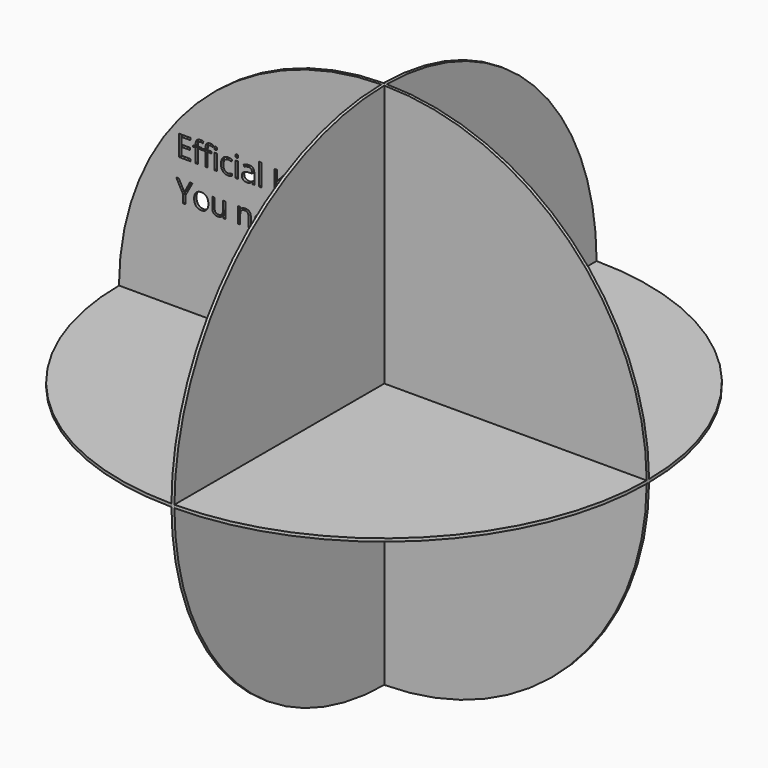
from build123d import *

# Parameters (mm, degrees)
F1_W          = 0.6405815172
F1_H          = 4.2273443089
F1_H_2        = 6.002211788
F2_DEPTH      = 0.4064
F2_DEPTH_BACK = 0.4064
F4_DEPTH      = 0.4064
F4_DEPTH_BACK = 0.4064
F6_DEPTH      = 0.4064
F6_DEPTH_BACK = 0.4064


# Not quite as in the source:
# - a variable given as a bare number and used for a length is read in inches; the dataset says mm whatever the document's units were
# - ends of sketch curves that miss each other by under 0.0002 mm in the source are joined


with BuildPart() as f2:
    # F1 (on Front) → F2 (new body, two sides)
    with BuildSketch(Plane.XZ) as f2_sk:
        with BuildLine():
            Line((35.941, 0.4064), (71.8808511569, 0.4064))
            ThreePointArc((71.8808511569, 0.4064), (0, 71.882), (-71.8808511569, 0.4064))
            Line((-71.8808511569, 0.4064), (-35.941, 0.4064))
            Line((-35.941, 0.4064), (-35.941, -0.4064))
            Line((-35.941, -0.4064), (-71.8808511569, -0.4064))
            ThreePointArc((-71.8808511569, -0.4064), (-50.8282496453, -50.8282496453), (-0.4064, -71.8808511569))
            Line((-0.4064, -71.8808511569), (-0.4064, 0))
            Line((-0.4064, 0), (0.4064, 0))
            Line((0.4064, 0), (0.4064, -71.8808511569))
            ThreePointArc((0.4064, -71.8808511569), (50.8282496453, -50.8282496453), (71.8808511569, -0.4064))
            Line((71.8808511569, -0.4064), (35.941, -0.4064))
            Line((35.941, -0.4064), (35.941, 0.4064))
        make_face()
        Polygon((-55.5503898714, 31.4164388821), (-54.0569339258, 28.596152241), (-52.5536038913, 31.4164388821), (-51.8439037518, 31.4164388821), (-53.7261519478, 27.9642105516), (-53.7261519478, 25.777099861), (-54.3889501649, 25.777099861), (-54.3889501649, 27.9333540238), (-56.2674955775, 31.4164388821), align=None, mode=Mode.SUBTRACT)
        with BuildLine():
            add(Edge.make_bspline(
                [(-48.0392938738, 29.4916086778), (-47.5165842929, 28.9010147357), (-47.5165842929, 27.8950919294)],
                knots=[0, 0, 0, 1, 1, 1], degree=2))
            add(Edge.make_bspline(
                [(-47.5165842929, 27.8950919294), (-47.5165842929, 26.8607811174), (-48.0368253516, 26.2800612642)],
                knots=[0, 0, 0, 1, 1, 1], degree=2))
            add(Edge.make_bspline(
                [(-48.0368253516, 26.2800612642), (-48.5570664104, 25.699341411), (-49.4753566778, 25.699341411)],
                knots=[0, 0, 0, 1, 1, 1], degree=2))
            add(Edge.make_bspline(
                [(-49.4753566778, 25.699341411), (-50.0431167893, 25.699341411), (-50.4825137452, 25.9659418112)],
                knots=[0, 0, 0, 1, 1, 1], degree=2))
            add(Edge.make_bspline(
                [(-50.4825137452, 25.9659418112), (-50.9219107011, 26.2325422114), (-51.1613573569, 26.7299494396)],
                knots=[0, 0, 0, 1, 1, 1], degree=2))
            add(Edge.make_bspline(
                [(-51.1613573569, 26.7299494396), (-51.4008040126, 27.2273566677), (-51.4008040126, 27.8950919294)],
                knots=[0, 0, 0, 1, 1, 1], degree=2))
            add(Edge.make_bspline(
                [(-51.4008040126, 27.8950919294), (-51.4008040126, 28.9281684802), (-50.8836486066, 29.5051855501)],
                knots=[0, 0, 0, 1, 1, 1], degree=2))
            add(Edge.make_bspline(
                [(-50.8836486066, 29.5051855501), (-50.3664932007, 30.08220262), (-49.4482029333, 30.08220262)],
                knots=[0, 0, 0, 1, 1, 1], degree=2))
            add(Edge.make_bspline(
                [(-49.4482029333, 30.08220262), (-48.5620034548, 30.08220262), (-48.0392938738, 29.4916086778)],
                knots=[0, 0, 0, 1, 1, 1], degree=2))
        make_face(mode=Mode.SUBTRACT)
        with BuildLine():
            Line((-46.439074342, 30.0044441699), (-45.7910872582, 30.0044441699))
            Line((-45.7910872582, 30.0044441699), (-45.7910872582, 27.2619159789))
            add(Edge.make_bspline(
                [(-45.7910872582, 27.2619159789), (-45.7910872582, 26.7447605729), (-45.5559605163, 26.4905027838)],
                knots=[0, 0, 0, 1, 1, 1], degree=2))
            add(Edge.make_bspline(
                [(-45.5559605163, 26.4905027838), (-45.3208337745, 26.2362449947), (-44.819723763, 26.2362449947)],
                knots=[0, 0, 0, 1, 1, 1], degree=2))
            add(Edge.make_bspline(
                [(-44.819723763, 26.2362449947), (-44.1556912847, 26.2362449947), (-43.8495945289, 26.5985006311)],
                knots=[0, 0, 0, 1, 1, 1], degree=2))
            add(Edge.make_bspline(
                [(-43.8495945289, 26.5985006311), (-43.5434977731, 26.9607562675), (-43.5434977731, 27.7827741682)],
                knots=[0, 0, 0, 1, 1, 1], degree=2))
            Line((-43.5434977731, 27.7827741682), (-43.5434977731, 30.0044441699))
            Line((-43.5434977731, 30.0044441699), (-42.9029162559, 30.0044441699))
            Line((-42.9029162559, 30.0044441699), (-42.9029162559, 25.777099861))
            Line((-42.9029162559, 25.777099861), (-43.4311800119, 25.777099861))
            Line((-43.4311800119, 25.777099861), (-43.5237495953, 26.3436257115))
            Line((-43.5237495953, 26.3436257115), (-43.5583089064, 26.3436257115))
            add(Edge.make_bspline(
                [(-43.5583089064, 26.3436257115), (-43.7545564233, 26.0313576501), (-44.103852318, 25.8653495306)],
                knots=[0, 0, 0, 1, 1, 1], degree=2))
            add(Edge.make_bspline(
                [(-44.103852318, 25.8653495306), (-44.4531482127, 25.699341411), (-44.9011849964, 25.699341411)],
                knots=[0, 0, 0, 1, 1, 1], degree=2))
            add(Edge.make_bspline(
                [(-44.9011849964, 25.699341411), (-45.6725981914, 25.699341411), (-46.0558362667, 26.0659169613)],
                knots=[0, 0, 0, 1, 1, 1], degree=2))
            add(Edge.make_bspline(
                [(-46.0558362667, 26.0659169613), (-46.439074342, 26.4324925116), (-46.439074342, 27.2384650177)],
                knots=[0, 0, 0, 1, 1, 1], degree=2))
            Line((-46.439074342, 27.2384650177), (-46.439074342, 30.0044441699))
        make_face(mode=Mode.SUBTRACT)
        with BuildLine():
            Line((-35.9589632394, 25.777099861), (-36.5995447565, 25.777099861))
            Line((-36.5995447565, 25.777099861), (-36.5995447565, 28.5122224854))
            add(Edge.make_bspline(
                [(-36.5995447565, 28.5122224854), (-36.5995447565, 29.0281436303), (-36.8346714984, 29.2830185499)],
                knots=[0, 0, 0, 1, 1, 1], degree=2))
            add(Edge.make_bspline(
                [(-36.8346714984, 29.2830185499), (-37.0697982402, 29.5378934695), (-37.5721425128, 29.5378934695)],
                knots=[0, 0, 0, 1, 1, 1], degree=2))
            add(Edge.make_bspline(
                [(-37.5721425128, 29.5378934695), (-38.23494073, 29.5378934695), (-38.5435060081, 29.1793406165)],
                knots=[0, 0, 0, 1, 1, 1], degree=2))
            add(Edge.make_bspline(
                [(-38.5435060081, 29.1793406165), (-38.8520712861, 28.8207877634), (-38.8520712861, 27.9950670794)],
                knots=[0, 0, 0, 1, 1, 1], degree=2))
            Line((-38.8520712861, 27.9950670794), (-38.8520712861, 25.777099861))
            Line((-38.8520712861, 25.777099861), (-39.4926528032, 25.777099861))
            Line((-39.4926528032, 25.777099861), (-39.4926528032, 30.0044441699))
            Line((-39.4926528032, 30.0044441699), (-38.9717946139, 30.0044441699))
            Line((-38.9717946139, 30.0044441699), (-38.8681166805, 29.4255757083))
            Line((-38.8681166805, 29.4255757083), (-38.8372601527, 29.4255757083))
            add(Edge.make_bspline(
                [(-38.8372601527, 29.4255757083), (-38.6397783748, 29.7378437697), (-38.2849283051, 29.9100231948)],
                knots=[0, 0, 0, 1, 1, 1], degree=2))
            add(Edge.make_bspline(
                [(-38.2849283051, 29.9100231948), (-37.9300782354, 30.08220262), (-37.4943840628, 30.08220262)],
                knots=[0, 0, 0, 1, 1, 1], degree=2))
            add(Edge.make_bspline(
                [(-37.4943840628, 30.08220262), (-36.7303764344, 30.08220262), (-36.3446698369, 29.713775678)],
                knots=[0, 0, 0, 1, 1, 1], degree=2))
            add(Edge.make_bspline(
                [(-36.3446698369, 29.713775678), (-35.9589632394, 29.3453487361), (-35.9589632394, 28.5344391854)],
                knots=[0, 0, 0, 1, 1, 1], degree=2))
            Line((-35.9589632394, 28.5344391854), (-35.9589632394, 25.777099861))
        make_face(mode=Mode.SUBTRACT)
        with BuildLine():
            add(Edge.make_bspline(
                [(-31.5187088886, 29.4916086778), (-30.9959993077, 28.9010147357), (-30.9959993077, 27.8950919294)],
                knots=[0, 0, 0, 1, 1, 1], degree=2))
            add(Edge.make_bspline(
                [(-30.9959993077, 27.8950919294), (-30.9959993077, 26.8607811174), (-31.5162403664, 26.2800612642)],
                knots=[0, 0, 0, 1, 1, 1], degree=2))
            add(Edge.make_bspline(
                [(-31.5162403664, 26.2800612642), (-32.0364814252, 25.699341411), (-32.9547716926, 25.699341411)],
                knots=[0, 0, 0, 1, 1, 1], degree=2))
            add(Edge.make_bspline(
                [(-32.9547716926, 25.699341411), (-33.5225318041, 25.699341411), (-33.96192876, 25.9659418112)],
                knots=[0, 0, 0, 1, 1, 1], degree=2))
            add(Edge.make_bspline(
                [(-33.96192876, 25.9659418112), (-34.4013257159, 26.2325422114), (-34.6407723717, 26.7299494396)],
                knots=[0, 0, 0, 1, 1, 1], degree=2))
            add(Edge.make_bspline(
                [(-34.6407723717, 26.7299494396), (-34.8802190274, 27.2273566677), (-34.8802190274, 27.8950919294)],
                knots=[0, 0, 0, 1, 1, 1], degree=2))
            add(Edge.make_bspline(
                [(-34.8802190274, 27.8950919294), (-34.8802190274, 28.9281684802), (-34.3630636214, 29.5051855501)],
                knots=[0, 0, 0, 1, 1, 1], degree=2))
            add(Edge.make_bspline(
                [(-34.3630636214, 29.5051855501), (-33.8459082155, 30.08220262), (-32.9276179481, 30.08220262)],
                knots=[0, 0, 0, 1, 1, 1], degree=2))
            add(Edge.make_bspline(
                [(-32.9276179481, 30.08220262), (-32.0414184696, 30.08220262), (-31.5187088886, 29.4916086778)],
                knots=[0, 0, 0, 1, 1, 1], degree=2))
        make_face(mode=Mode.SUBTRACT)
        with BuildLine():
            add(Edge.make_bspline(
                [(-29.0051361339, 26.4331096421), (-28.8236997504, 26.2288394281), (-28.5077289057, 26.2288394281)],
                knots=[0, 0, 0, 1, 1, 1], degree=2))
            add(Edge.make_bspline(
                [(-28.5077289057, 26.2288394281), (-28.3374008723, 26.2288394281), (-28.1794154499, 26.2535246503)],
                knots=[0, 0, 0, 1, 1, 1], degree=2))
            add(Edge.make_bspline(
                [(-28.1794154499, 26.2535246503), (-28.0214300276, 26.2782098725), (-27.9288604442, 26.305363617)],
                knots=[0, 0, 0, 1, 1, 1], degree=2))
            Line((-27.9288604442, 26.305363617), (-27.9288604442, 25.8153619555))
            add(Edge.make_bspline(
                [(-27.9288604442, 25.8153619555), (-28.0325383776, 25.765991511), (-28.2349572, 25.732666461)],
                knots=[0, 0, 0, 1, 1, 1], degree=2))
            add(Edge.make_bspline(
                [(-28.2349572, 25.732666461), (-28.4373760223, 25.699341411), (-28.6002984891, 25.699341411)],
                knots=[0, 0, 0, 1, 1, 1], degree=2))
            add(Edge.make_bspline(
                [(-28.6002984891, 25.699341411), (-29.8259197734, 25.699341411), (-29.8259197734, 26.9916127953)],
                knots=[0, 0, 0, 1, 1, 1], degree=2))
            Line((-29.8259197734, 26.9916127953), (-29.8259197734, 29.5070369417))
            Line((-29.8259197734, 29.5070369417), (-30.4319419795, 29.5070369417))
            Line((-30.4319419795, 29.5070369417), (-30.4319419795, 29.8156022198))
            Line((-30.4319419795, 29.8156022198), (-29.8259197734, 30.08220262))
            Line((-29.8259197734, 30.08220262), (-29.556850851, 30.9844474929))
            Line((-29.556850851, 30.9844474929), (-29.1865725174, 30.9844474929))
            Line((-29.1865725174, 30.9844474929), (-29.1865725174, 30.0044441699))
            Line((-29.1865725174, 30.0044441699), (-27.959716972, 30.0044441699))
            Line((-27.959716972, 30.0044441699), (-27.959716972, 29.5070369417))
            Line((-27.959716972, 29.5070369417), (-29.1865725174, 29.5070369417))
            Line((-29.1865725174, 29.5070369417), (-29.1865725174, 27.0187665398))
            add(Edge.make_bspline(
                [(-29.1865725174, 27.0187665398), (-29.1865725174, 26.6373798562), (-29.0051361339, 26.4331096421)],
                knots=[0, 0, 0, 1, 1, 1], degree=2))
        make_face(mode=Mode.SUBTRACT)
        with BuildLine():
            Line((-25.0777172753, 30.0044441699), (-24.4297301914, 30.0044441699))
            Line((-24.4297301914, 30.0044441699), (-24.4297301914, 27.2619159789))
            add(Edge.make_bspline(
                [(-24.4297301914, 27.2619159789), (-24.4297301914, 26.7447605729), (-24.1946034496, 26.4905027838)],
                knots=[0, 0, 0, 1, 1, 1], degree=2))
            add(Edge.make_bspline(
                [(-24.1946034496, 26.4905027838), (-23.9594767077, 26.2362449947), (-23.4583666962, 26.2362449947)],
                knots=[0, 0, 0, 1, 1, 1], degree=2))
            add(Edge.make_bspline(
                [(-23.4583666962, 26.2362449947), (-22.7943342179, 26.2362449947), (-22.4882374621, 26.5985006311)],
                knots=[0, 0, 0, 1, 1, 1], degree=2))
            add(Edge.make_bspline(
                [(-22.4882374621, 26.5985006311), (-22.1821407063, 26.9607562675), (-22.1821407063, 27.7827741682)],
                knots=[0, 0, 0, 1, 1, 1], degree=2))
            Line((-22.1821407063, 27.7827741682), (-22.1821407063, 30.0044441699))
            Line((-22.1821407063, 30.0044441699), (-21.5415591891, 30.0044441699))
            Line((-21.5415591891, 30.0044441699), (-21.5415591891, 25.777099861))
            Line((-21.5415591891, 25.777099861), (-22.0698229451, 25.777099861))
            Line((-22.0698229451, 25.777099861), (-22.1623925285, 26.3436257115))
            Line((-22.1623925285, 26.3436257115), (-22.1969518397, 26.3436257115))
            add(Edge.make_bspline(
                [(-22.1969518397, 26.3436257115), (-22.3931993565, 26.0313576501), (-22.7424952512, 25.8653495306)],
                knots=[0, 0, 0, 1, 1, 1], degree=2))
            add(Edge.make_bspline(
                [(-22.7424952512, 25.8653495306), (-23.0917911459, 25.699341411), (-23.5398279296, 25.699341411)],
                knots=[0, 0, 0, 1, 1, 1], degree=2))
            add(Edge.make_bspline(
                [(-23.5398279296, 25.699341411), (-24.3112411247, 25.699341411), (-24.6944792, 26.0659169613)],
                knots=[0, 0, 0, 1, 1, 1], degree=2))
            add(Edge.make_bspline(
                [(-24.6944792, 26.0659169613), (-25.0777172753, 26.4324925116), (-25.0777172753, 27.2384650177)],
                knots=[0, 0, 0, 1, 1, 1], degree=2))
            Line((-25.0777172753, 27.2384650177), (-25.0777172753, 30.0044441699))
        make_face(mode=Mode.SUBTRACT)
        with BuildLine():
            add(Edge.make_bspline(
                [(-16.9260397605, 26.2763584809), (-17.3907390692, 25.699341411), (-18.2164597532, 25.699341411)],
                knots=[0, 0, 0, 1, 1, 1], degree=2))
            add(Edge.make_bspline(
                [(-18.2164597532, 25.699341411), (-18.6299372257, 25.699341411), (-18.9712104232, 25.8517726583)],
                knots=[0, 0, 0, 1, 1, 1], degree=2))
            add(Edge.make_bspline(
                [(-18.9712104232, 25.8517726583), (-19.3124836207, 26.0042039057), (-19.5432904487, 26.3214090115)],
                knots=[0, 0, 0, 1, 1, 1], degree=2))
            Line((-19.5432904487, 26.3214090115), (-19.5901923709, 26.3214090115))
            add(Edge.make_bspline(
                [(-19.5901923709, 26.3214090115), (-19.5432904487, 25.9511306778), (-19.5432904487, 25.6191144387)],
                knots=[0, 0, 0, 1, 1, 1], degree=2))
            Line((-19.5432904487, 25.6191144387), (-19.5432904487, 23.8788062707))
            Line((-19.5432904487, 23.8788062707), (-20.1838719659, 23.8788062707))
            Line((-20.1838719659, 23.8788062707), (-20.1838719659, 30.0044441699))
            Line((-20.1838719659, 30.0044441699), (-19.6630137766, 30.0044441699))
            Line((-19.6630137766, 30.0044441699), (-19.5741469765, 29.4255757083))
            Line((-19.5741469765, 29.4255757083), (-19.5432904487, 29.4255757083))
            add(Edge.make_bspline(
                [(-19.5432904487, 29.4255757083), (-19.2964382263, 29.773637342), (-18.968741901, 29.927919981)],
                knots=[0, 0, 0, 1, 1, 1], degree=2))
            add(Edge.make_bspline(
                [(-18.968741901, 29.927919981), (-18.6410455758, 30.08220262), (-18.2164597532, 30.08220262)],
                knots=[0, 0, 0, 1, 1, 1], degree=2))
            add(Edge.make_bspline(
                [(-18.2164597532, 30.08220262), (-17.3759279359, 30.08220262), (-16.9186341938, 29.5070369417)],
                knots=[0, 0, 0, 1, 1, 1], degree=2))
            add(Edge.make_bspline(
                [(-16.9186341938, 29.5070369417), (-16.4613404518, 28.9318712635), (-16.4613404518, 27.8950919294)],
                knots=[0, 0, 0, 1, 1, 1], degree=2))
            add(Edge.make_bspline(
                [(-16.4613404518, 27.8950919294), (-16.4613404518, 26.8533755508), (-16.9260397605, 26.2763584809)],
                knots=[0, 0, 0, 1, 1, 1], degree=2))
        make_face(mode=Mode.SUBTRACT)
        with BuildLine():
            add(Edge.make_bspline(
                [(-14.9647988534, 25.7863568194), (-15.0962476619, 25.9079315389), (-15.0962476619, 26.1856402891)],
                knots=[0, 0, 0, 1, 1, 1], degree=2))
            add(Edge.make_bspline(
                [(-15.0962476619, 26.1856402891), (-15.0962476619, 26.7102012618), (-14.6333997448, 26.7102012618)],
                knots=[0, 0, 0, 1, 1, 1], degree=2))
            add(Edge.make_bspline(
                [(-14.6333997448, 26.7102012618), (-14.4099984835, 26.7102012618), (-14.288423764, 26.5756668006)],
                knots=[0, 0, 0, 1, 1, 1], degree=2))
            add(Edge.make_bspline(
                [(-14.288423764, 26.5756668006), (-14.1668490445, 26.4411323393), (-14.1668490445, 26.1856402891)],
                knots=[0, 0, 0, 1, 1, 1], degree=2))
            add(Edge.make_bspline(
                [(-14.1668490445, 26.1856402891), (-14.1668490445, 25.9387880667), (-14.2902751557, 25.8017850833)],
                knots=[0, 0, 0, 1, 1, 1], degree=2))
            add(Edge.make_bspline(
                [(-14.2902751557, 25.8017850833), (-14.4137012669, 25.6647820998), (-14.6333997448, 25.6647820998)],
                knots=[0, 0, 0, 1, 1, 1], degree=2))
            add(Edge.make_bspline(
                [(-14.6333997448, 25.6647820998), (-14.833350045, 25.6647820998), (-14.9647988534, 25.7863568194)],
                knots=[0, 0, 0, 1, 1, 1], degree=2))
        make_face(mode=Mode.SUBTRACT)
        with BuildLine():
            Line((-14.4099984835, 27.3310346011), (-14.9074057117, 27.3310346011))
            Line((-14.9074057117, 27.3310346011), (-14.9074057117, 27.5396247291))
            add(Edge.make_bspline(
                [(-14.9074057117, 27.5396247291), (-14.9074057117, 27.9913642961), (-14.7685513366, 28.2826499186)],
                knots=[0, 0, 0, 1, 1, 1], degree=2))
            add(Edge.make_bspline(
                [(-14.7685513366, 28.2826499186), (-14.6296969615, 28.573935541), (-14.2520130612, 28.8973119524)],
                knots=[0, 0, 0, 1, 1, 1], degree=2))
            add(Edge.make_bspline(
                [(-14.2520130612, 28.8973119524), (-13.7274520886, 29.3416459527), (-13.5904491051, 29.565047214)],
                knots=[0, 0, 0, 1, 1, 1], degree=2))
            add(Edge.make_bspline(
                [(-13.5904491051, 29.565047214), (-13.4534461217, 29.7884484753), (-13.4534461217, 30.10441932)],
                knots=[0, 0, 0, 1, 1, 1], degree=2))
            add(Edge.make_bspline(
                [(-13.4534461217, 30.10441932), (-13.4534461217, 30.4981486147), (-13.7058525191, 30.7122929177)],
                knots=[0, 0, 0, 1, 1, 1], degree=2))
            add(Edge.make_bspline(
                [(-13.7058525191, 30.7122929177), (-13.9582589165, 30.9264372206), (-14.4322151836, 30.9264372206)],
                knots=[0, 0, 0, 1, 1, 1], degree=2))
            add(Edge.make_bspline(
                [(-14.4322151836, 30.9264372206), (-14.7370776782, 30.9264372206), (-15.026511909, 30.8548500761)],
                knots=[0, 0, 0, 1, 1, 1], degree=2))
            add(Edge.make_bspline(
                [(-15.026511909, 30.8548500761), (-15.3159461398, 30.7832629316), (-15.6899272568, 30.5944209815)],
                knots=[0, 0, 0, 1, 1, 1], degree=2))
            Line((-15.6899272568, 30.5944209815), (-15.9182655625, 31.1152791708))
            add(Edge.make_bspline(
                [(-15.9182655625, 31.1152791708), (-15.1888172453, 31.4966658544), (-14.3939530891, 31.4966658544)],
                knots=[0, 0, 0, 1, 1, 1], degree=2))
            add(Edge.make_bspline(
                [(-14.3939530891, 31.4966658544), (-13.6570992052, 31.4966658544), (-13.2485587771, 31.134410218)],
                knots=[0, 0, 0, 1, 1, 1], degree=2))
            add(Edge.make_bspline(
                [(-13.2485587771, 31.134410218), (-12.840018349, 30.7721545816), (-12.840018349, 30.1130591478)],
                knots=[0, 0, 0, 1, 1, 1], degree=2))
            add(Edge.make_bspline(
                [(-12.840018349, 30.1130591478), (-12.840018349, 29.8304133531), (-12.9153082768, 29.6168861807)],
                knots=[0, 0, 0, 1, 1, 1], degree=2))
            add(Edge.make_bspline(
                [(-12.9153082768, 29.6168861807), (-12.9905982046, 29.4033590083), (-13.1368581464, 29.212048536)],
                knots=[0, 0, 0, 1, 1, 1], degree=2))
            add(Edge.make_bspline(
                [(-13.1368581464, 29.212048536), (-13.2831180882, 29.0207380636), (-13.7694169664, 28.596152241)],
                knots=[0, 0, 0, 1, 1, 1], degree=2))
            add(Edge.make_bspline(
                [(-13.7694169664, 28.596152241), (-14.1594434778, 28.265370263), (-14.2847209807, 28.0450546545)],
                knots=[0, 0, 0, 1, 1, 1], degree=2))
            add(Edge.make_bspline(
                [(-14.2847209807, 28.0450546545), (-14.4099984835, 27.824739046), (-14.4099984835, 27.4593977568)],
                knots=[0, 0, 0, 1, 1, 1], degree=2))
            Line((-14.4099984835, 27.4593977568), (-14.4099984835, 27.3310346011))
        make_face(mode=Mode.SUBTRACT)
        Polygon((-52.3487165467, 37.1063826088), (-52.3487165467, 36.5201085806), (-55.4923795991, 36.5201085806), (-55.4923795991, 42.1594476017), (-52.3487165467, 42.1594476017), (-52.3487165467, 41.5768763568), (-54.8369869486, 41.5768763568), (-54.8369869486, 39.7600439998), (-52.4992964024, 39.7600439998), (-52.4992964024, 39.1811755382), (-54.8369869486, 39.1811755382), (-54.8369869486, 37.1063826088), align=None, mode=Mode.SUBTRACT)
        with BuildLine():
            Line((-49.2902175109, 40.7474528895), (-49.2902175109, 40.2500456613))
            Line((-49.2902175109, 40.2500456613), (-50.3664932007, 40.2500456613))
            Line((-50.3664932007, 40.2500456613), (-50.3664932007, 36.5201085806))
            Line((-50.3664932007, 36.5201085806), (-51.0070747178, 36.5201085806))
            Line((-51.0070747178, 36.5201085806), (-51.0070747178, 40.2500456613))
            Line((-51.0070747178, 40.2500456613), (-51.7624425184, 40.2500456613))
            Line((-51.7624425184, 40.2500456613), (-51.7624425184, 40.5388627615))
            Line((-51.7624425184, 40.5388627615), (-51.0070747178, 40.7709038506))
            Line((-51.0070747178, 40.7709038506), (-51.0070747178, 41.0054134619))
            add(Edge.make_bspline(
                [(-51.0070747178, 41.0054134619), (-51.0070747178, 42.5642852464), (-49.6456847112, 42.5642852464)],
                knots=[0, 0, 0, 1, 1, 1], degree=2))
            add(Edge.make_bspline(
                [(-49.6456847112, 42.5642852464), (-49.3099656887, 42.5642852464), (-48.8582261217, 42.4297507852)],
                knots=[0, 0, 0, 1, 1, 1], degree=2))
            Line((-48.8582261217, 42.4297507852), (-49.0248513718, 41.9162981626))
            add(Edge.make_bspline(
                [(-49.0248513718, 41.9162981626), (-49.3951297055, 42.0360214905), (-49.6567930612, 42.0360214905)],
                knots=[0, 0, 0, 1, 1, 1], degree=2))
            add(Edge.make_bspline(
                [(-49.6567930612, 42.0360214905), (-50.0196658282, 42.0360214905), (-50.1930795144, 41.7947234431)],
                knots=[0, 0, 0, 1, 1, 1], degree=2))
            add(Edge.make_bspline(
                [(-50.1930795144, 41.7947234431), (-50.3664932007, 41.5534253957), (-50.3664932007, 41.0214588563)],
                knots=[0, 0, 0, 1, 1, 1], degree=2))
            Line((-50.3664932007, 41.0214588563), (-50.3664932007, 40.7474528895))
            Line((-50.3664932007, 40.7474528895), (-49.2902175109, 40.7474528895))
        make_face(mode=Mode.SUBTRACT)
        with BuildLine():
            Line((-46.6131051588, 40.7474528895), (-46.6131051588, 40.2500456613))
            Line((-46.6131051588, 40.2500456613), (-47.6893808486, 40.2500456613))
            Line((-47.6893808486, 40.2500456613), (-47.6893808486, 36.5201085806))
            Line((-47.6893808486, 36.5201085806), (-48.3299623657, 36.5201085806))
            Line((-48.3299623657, 36.5201085806), (-48.3299623657, 40.2500456613))
            Line((-48.3299623657, 40.2500456613), (-49.0853301663, 40.2500456613))
            Line((-49.0853301663, 40.2500456613), (-49.0853301663, 40.5388627615))
            Line((-49.0853301663, 40.5388627615), (-48.3299623657, 40.7709038506))
            Line((-48.3299623657, 40.7709038506), (-48.3299623657, 41.0054134619))
            add(Edge.make_bspline(
                [(-48.3299623657, 41.0054134619), (-48.3299623657, 42.5642852464), (-46.9685723591, 42.5642852464)],
                knots=[0, 0, 0, 1, 1, 1], degree=2))
            add(Edge.make_bspline(
                [(-46.9685723591, 42.5642852464), (-46.6328533366, 42.5642852464), (-46.1811137696, 42.4297507852)],
                knots=[0, 0, 0, 1, 1, 1], degree=2))
            Line((-46.1811137696, 42.4297507852), (-46.3477390197, 41.9162981626))
            add(Edge.make_bspline(
                [(-46.3477390197, 41.9162981626), (-46.7180173534, 42.0360214905), (-46.9796807091, 42.0360214905)],
                knots=[0, 0, 0, 1, 1, 1], degree=2))
            add(Edge.make_bspline(
                [(-46.9796807091, 42.0360214905), (-47.3425534761, 42.0360214905), (-47.5159671623, 41.7947234431)],
                knots=[0, 0, 0, 1, 1, 1], degree=2))
            add(Edge.make_bspline(
                [(-47.5159671623, 41.7947234431), (-47.6893808486, 41.5534253957), (-47.6893808486, 41.0214588563)],
                knots=[0, 0, 0, 1, 1, 1], degree=2))
            Line((-47.6893808486, 41.0214588563), (-47.6893808486, 40.7474528895))
            Line((-47.6893808486, 40.7474528895), (-46.6131051588, 40.7474528895))
        make_face(mode=Mode.SUBTRACT)
        with Locations((-45.5214012052, 38.633780735)):
            Rectangle(F1_W, F1_H, mode=Mode.SUBTRACT)
        with BuildLine():
            add(Edge.make_bspline(
                [(-45.7880016054, 41.5707050512), (-45.8959994527, 41.6768515069), (-45.8959994527, 41.8928472015)],
                knots=[0, 0, 0, 1, 1, 1], degree=2))
            add(Edge.make_bspline(
                [(-45.8959994527, 41.8928472015), (-45.8959994527, 42.1125456794), (-45.7880016054, 42.2149893517)],
                knots=[0, 0, 0, 1, 1, 1], degree=2))
            add(Edge.make_bspline(
                [(-45.7880016054, 42.2149893517), (-45.6800037581, 42.317433024), (-45.5170812913, 42.317433024)],
                knots=[0, 0, 0, 1, 1, 1], degree=2))
            add(Edge.make_bspline(
                [(-45.5170812913, 42.317433024), (-45.3627986523, 42.317433024), (-45.2510980217, 42.2131379601)],
                knots=[0, 0, 0, 1, 1, 1], degree=2))
            add(Edge.make_bspline(
                [(-45.2510980217, 42.2131379601), (-45.139397391, 42.1088428961), (-45.139397391, 41.8928472015)],
                knots=[0, 0, 0, 1, 1, 1], degree=2))
            add(Edge.make_bspline(
                [(-45.139397391, 41.8928472015), (-45.139397391, 41.6768515069), (-45.2510980217, 41.5707050512)],
                knots=[0, 0, 0, 1, 1, 1], degree=2))
            add(Edge.make_bspline(
                [(-45.2510980217, 41.5707050512), (-45.3627986523, 41.4645585956), (-45.5170812913, 41.4645585956)],
                knots=[0, 0, 0, 1, 1, 1], degree=2))
            add(Edge.make_bspline(
                [(-45.5170812913, 41.4645585956), (-45.6800037581, 41.4645585956), (-45.7880016054, 41.5707050512)],
                knots=[0, 0, 0, 1, 1, 1], degree=2))
        make_face(mode=Mode.SUBTRACT)
        with BuildLine():
            add(Edge.make_bspline(
                [(-41.0860838989, 36.6632828696), (-41.5094354604, 36.4423501305), (-42.1537197609, 36.4423501305)],
                knots=[0, 0, 0, 1, 1, 1], degree=2))
            add(Edge.make_bspline(
                [(-42.1537197609, 36.4423501305), (-43.0720100283, 36.4423501305), (-43.575588562, 37.0076417199)],
                knots=[0, 0, 0, 1, 1, 1], degree=2))
            add(Edge.make_bspline(
                [(-43.575588562, 37.0076417199), (-44.0791670957, 37.5729333092), (-44.0791670957, 38.6072441211)],
                knots=[0, 0, 0, 1, 1, 1], degree=2))
            add(Edge.make_bspline(
                [(-44.0791670957, 38.6072441211), (-44.0791670957, 39.6674744164), (-43.5675658648, 40.246342878)],
                knots=[0, 0, 0, 1, 1, 1], degree=2))
            add(Edge.make_bspline(
                [(-43.5675658648, 40.246342878), (-43.0559646338, 40.8252113395), (-42.1117548831, 40.8252113395)],
                knots=[0, 0, 0, 1, 1, 1], degree=2))
            add(Edge.make_bspline(
                [(-42.1117548831, 40.8252113395), (-41.8068923884, 40.8252113395), (-41.5020298937, 40.75917837)],
                knots=[0, 0, 0, 1, 1, 1], degree=2))
            add(Edge.make_bspline(
                [(-41.5020298937, 40.75917837), (-41.197167399, 40.6931454005), (-41.0243708433, 40.6042786005)],
                knots=[0, 0, 0, 1, 1, 1], degree=2))
            Line((-41.0243708433, 40.6042786005), (-41.2206183602, 40.0612037111))
            add(Edge.make_bspline(
                [(-41.2206183602, 40.0612037111), (-41.4329112714, 40.1463677279), (-41.6834662772, 40.2019094779)],
                knots=[0, 0, 0, 1, 1, 1], degree=2))
            add(Edge.make_bspline(
                [(-41.6834662772, 40.2019094779), (-41.9340212829, 40.257451228), (-42.1265660164, 40.257451228)],
                knots=[0, 0, 0, 1, 1, 1], degree=2))
            add(Edge.make_bspline(
                [(-42.1265660164, 40.257451228), (-43.4151346174, 40.257451228), (-43.4151346174, 38.6146496878)],
                knots=[0, 0, 0, 1, 1, 1], degree=2))
            add(Edge.make_bspline(
                [(-43.4151346174, 38.6146496878), (-43.4151346174, 37.8358309261), (-43.1010151644, 37.4192678007)],
                knots=[0, 0, 0, 1, 1, 1], degree=2))
            add(Edge.make_bspline(
                [(-43.1010151644, 37.4192678007), (-42.7868957114, 37.0027046754), (-42.1697651553, 37.0027046754)],
                knots=[0, 0, 0, 1, 1, 1], degree=2))
            add(Edge.make_bspline(
                [(-42.1697651553, 37.0027046754), (-41.6415013994, 37.0027046754), (-41.0860838989, 37.22980872)],
                knots=[0, 0, 0, 1, 1, 1], degree=2))
            Line((-41.0860838989, 37.22980872), (-41.0860838989, 36.6632828696))
        make_face(mode=Mode.SUBTRACT)
        with Locations((-39.7623388562, 38.633780735)):
            Rectangle(F1_W, F1_H, mode=Mode.SUBTRACT)
        with BuildLine():
            Line((-35.0098164442, 36.5201085806), (-35.4850069723, 36.5201085806))
            Line((-35.4850069723, 36.5201085806), (-35.6121358669, 37.1224280033))
            Line((-35.6121358669, 37.1224280033), (-35.6429923947, 37.1224280033))
            add(Edge.make_bspline(
                [(-35.6429923947, 37.1224280033), (-35.9589632394, 36.7249959252), (-36.2730826924, 36.5836730279)],
                knots=[0, 0, 0, 1, 1, 1], degree=2))
            add(Edge.make_bspline(
                [(-36.2730826924, 36.5836730279), (-36.5872021454, 36.4423501305), (-37.0586898902, 36.4423501305)],
                knots=[0, 0, 0, 1, 1, 1], degree=2))
            add(Edge.make_bspline(
                [(-37.0586898902, 36.4423501305), (-37.6869287963, 36.4423501305), (-38.0436302577, 36.766960803)],
                knots=[0, 0, 0, 1, 1, 1], degree=2))
            add(Edge.make_bspline(
                [(-38.0436302577, 36.766960803), (-38.4003317191, 37.0915714755), (-38.4003317191, 37.6889538537)],
                knots=[0, 0, 0, 1, 1, 1], degree=2))
            add(Edge.make_bspline(
                [(-38.4003317191, 37.6889538537), (-38.4003317191, 38.968882627), (-36.3526925341, 39.0305956826)],
                knots=[0, 0, 0, 1, 1, 1], degree=2))
            Line((-36.3526925341, 39.0305956826), (-35.635586828, 39.0540466437))
            Line((-35.635586828, 39.0540466437), (-35.635586828, 39.3169442606))
            add(Edge.make_bspline(
                [(-35.635586828, 39.3169442606), (-35.635586828, 39.8143514887), (-35.8491140004, 40.0513296223)],
                knots=[0, 0, 0, 1, 1, 1], degree=2))
            add(Edge.make_bspline(
                [(-35.8491140004, 40.0513296223), (-36.0626411728, 40.2883077558), (-36.5341289176, 40.2883077558)],
                knots=[0, 0, 0, 1, 1, 1], degree=2))
            add(Edge.make_bspline(
                [(-36.5341289176, 40.2883077558), (-37.0623926736, 40.2883077558), (-37.7288936741, 39.9649313444)],
                knots=[0, 0, 0, 1, 1, 1], degree=2))
            Line((-37.7288936741, 39.9649313444), (-37.926375452, 40.4549330059))
            add(Edge.make_bspline(
                [(-37.926375452, 40.4549330059), (-37.6141073907, 40.6240267783), (-37.2419776654, 40.720299145)],
                knots=[0, 0, 0, 1, 1, 1], degree=2))
            add(Edge.make_bspline(
                [(-37.2419776654, 40.720299145), (-36.8698479401, 40.8165715117), (-36.494632562, 40.8165715117)],
                knots=[0, 0, 0, 1, 1, 1], degree=2))
            add(Edge.make_bspline(
                [(-36.494632562, 40.8165715117), (-35.7392647614, 40.8165715117), (-35.3745406028, 40.4814696198)],
                knots=[0, 0, 0, 1, 1, 1], degree=2))
            add(Edge.make_bspline(
                [(-35.3745406028, 40.4814696198), (-35.0098164442, 40.1463677279), (-35.0098164442, 39.4058110606)],
                knots=[0, 0, 0, 1, 1, 1], degree=2))
            Line((-35.0098164442, 39.4058110606), (-35.0098164442, 36.5201085806))
        make_face(mode=Mode.SUBTRACT)
        with BuildLine():
            add(Edge.make_bspline(
                [(-40.0289392564, 41.5707050512), (-40.1369371038, 41.6768515069), (-40.1369371038, 41.8928472015)],
                knots=[0, 0, 0, 1, 1, 1], degree=2))
            add(Edge.make_bspline(
                [(-40.1369371038, 41.8928472015), (-40.1369371038, 42.1125456794), (-40.0289392564, 42.2149893517)],
                knots=[0, 0, 0, 1, 1, 1], degree=2))
            add(Edge.make_bspline(
                [(-40.0289392564, 42.2149893517), (-39.9209414091, 42.317433024), (-39.7580189423, 42.317433024)],
                knots=[0, 0, 0, 1, 1, 1], degree=2))
            add(Edge.make_bspline(
                [(-39.7580189423, 42.317433024), (-39.6037363033, 42.317433024), (-39.4920356727, 42.2131379601)],
                knots=[0, 0, 0, 1, 1, 1], degree=2))
            add(Edge.make_bspline(
                [(-39.4920356727, 42.2131379601), (-39.380335042, 42.1088428961), (-39.380335042, 41.8928472015)],
                knots=[0, 0, 0, 1, 1, 1], degree=2))
            add(Edge.make_bspline(
                [(-39.380335042, 41.8928472015), (-39.380335042, 41.6768515069), (-39.4920356727, 41.5707050512)],
                knots=[0, 0, 0, 1, 1, 1], degree=2))
            add(Edge.make_bspline(
                [(-39.4920356727, 41.5707050512), (-39.6037363033, 41.4645585956), (-39.7580189423, 41.4645585956)],
                knots=[0, 0, 0, 1, 1, 1], degree=2))
            add(Edge.make_bspline(
                [(-39.7580189423, 41.4645585956), (-39.9209414091, 41.4645585956), (-40.0289392564, 41.5707050512)],
                knots=[0, 0, 0, 1, 1, 1], degree=2))
        make_face(mode=Mode.SUBTRACT)
        with Locations((-33.3713348179, 39.5212144746)):
            Rectangle(F1_W, F1_H_2, mode=Mode.SUBTRACT)
        Polygon((-27.8239482496, 39.7094392942), (-25.47144657, 36.5201085806), (-26.2428597651, 36.5201085806), (-28.2979045167, 39.255231205), (-28.8891155894, 38.7306702323), (-28.8891155894, 36.5201085806), (-29.5445082399, 36.5201085806), (-29.5445082399, 42.1594476017), (-28.8891155894, 42.1594476017), (-28.8891155894, 39.3626119217), (-26.3317265651, 42.1594476017), (-25.5566105867, 42.1594476017), align=None, mode=Mode.SUBTRACT)
        with BuildLine():
            Line((-21.2589133945, 36.5201085806), (-21.8994949116, 36.5201085806))
            Line((-21.8994949116, 36.5201085806), (-21.8994949116, 39.255231205))
            add(Edge.make_bspline(
                [(-21.8994949116, 39.255231205), (-21.8994949116, 39.7711523498), (-22.1346216535, 40.0260272695)],
                knots=[0, 0, 0, 1, 1, 1], degree=2))
            add(Edge.make_bspline(
                [(-22.1346216535, 40.0260272695), (-22.3697483954, 40.2809021891), (-22.872092668, 40.2809021891)],
                knots=[0, 0, 0, 1, 1, 1], degree=2))
            add(Edge.make_bspline(
                [(-22.872092668, 40.2809021891), (-23.5348908852, 40.2809021891), (-23.8434561632, 39.922349336)],
                knots=[0, 0, 0, 1, 1, 1], degree=2))
            add(Edge.make_bspline(
                [(-23.8434561632, 39.922349336), (-24.1520214412, 39.563796483), (-24.1520214412, 38.738075799)],
                knots=[0, 0, 0, 1, 1, 1], degree=2))
            Line((-24.1520214412, 38.738075799), (-24.1520214412, 36.5201085806))
            Line((-24.1520214412, 36.5201085806), (-24.7926029584, 36.5201085806))
            Line((-24.7926029584, 36.5201085806), (-24.7926029584, 40.7474528895))
            Line((-24.7926029584, 40.7474528895), (-24.2717447691, 40.7474528895))
            Line((-24.2717447691, 40.7474528895), (-24.1680668357, 40.1685844279))
            Line((-24.1680668357, 40.1685844279), (-24.1372103078, 40.1685844279))
            add(Edge.make_bspline(
                [(-24.1372103078, 40.1685844279), (-23.9397285299, 40.4808524893), (-23.5848784602, 40.6530319144)],
                knots=[0, 0, 0, 1, 1, 1], degree=2))
            add(Edge.make_bspline(
                [(-23.5848784602, 40.6530319144), (-23.2300283905, 40.8252113395), (-22.7943342179, 40.8252113395)],
                knots=[0, 0, 0, 1, 1, 1], degree=2))
            add(Edge.make_bspline(
                [(-22.7943342179, 40.8252113395), (-22.0303265895, 40.8252113395), (-21.644619992, 40.4567843976)],
                knots=[0, 0, 0, 1, 1, 1], degree=2))
            add(Edge.make_bspline(
                [(-21.644619992, 40.4567843976), (-21.2589133945, 40.0883574556), (-21.2589133945, 39.277447905)],
                knots=[0, 0, 0, 1, 1, 1], degree=2))
            Line((-21.2589133945, 39.277447905), (-21.2589133945, 36.5201085806))
        make_face(mode=Mode.SUBTRACT)
        with BuildLine():
            add(Edge.make_bspline(
                [(-16.8186590438, 40.2346173974), (-16.2959494628, 39.6440234553), (-16.2959494628, 38.6381006489)],
                knots=[0, 0, 0, 1, 1, 1], degree=2))
            add(Edge.make_bspline(
                [(-16.2959494628, 38.6381006489), (-16.2959494628, 37.603789837), (-16.8161905215, 37.0230699838)],
                knots=[0, 0, 0, 1, 1, 1], degree=2))
            add(Edge.make_bspline(
                [(-16.8161905215, 37.0230699838), (-17.3364315803, 36.4423501305), (-18.2547218477, 36.4423501305)],
                knots=[0, 0, 0, 1, 1, 1], degree=2))
            add(Edge.make_bspline(
                [(-18.2547218477, 36.4423501305), (-18.8224819592, 36.4423501305), (-19.2618789151, 36.7089505307)],
                knots=[0, 0, 0, 1, 1, 1], degree=2))
            add(Edge.make_bspline(
                [(-19.2618789151, 36.7089505307), (-19.701275871, 36.9755509309), (-19.9407225268, 37.4729581591)],
                knots=[0, 0, 0, 1, 1, 1], degree=2))
            add(Edge.make_bspline(
                [(-19.9407225268, 37.4729581591), (-20.1801691825, 37.9703653873), (-20.1801691825, 38.6381006489)],
                knots=[0, 0, 0, 1, 1, 1], degree=2))
            add(Edge.make_bspline(
                [(-20.1801691825, 38.6381006489), (-20.1801691825, 39.6711771997), (-19.6630137766, 40.2481942696)],
                knots=[0, 0, 0, 1, 1, 1], degree=2))
            add(Edge.make_bspline(
                [(-19.6630137766, 40.2481942696), (-19.1458583706, 40.8252113395), (-18.2275681032, 40.8252113395)],
                knots=[0, 0, 0, 1, 1, 1], degree=2))
            add(Edge.make_bspline(
                [(-18.2275681032, 40.8252113395), (-17.3413686247, 40.8252113395), (-16.8186590438, 40.2346173974)],
                knots=[0, 0, 0, 1, 1, 1], degree=2))
        make_face(mode=Mode.SUBTRACT)
        with BuildLine():
            add(Edge.make_bspline(
                [(-14.305086289, 37.1761183617), (-14.1236499055, 36.9718481476), (-13.8076790608, 36.9718481476)],
                knots=[0, 0, 0, 1, 1, 1], degree=2))
            add(Edge.make_bspline(
                [(-13.8076790608, 36.9718481476), (-13.6373510274, 36.9718481476), (-13.479365605, 36.9965333699)],
                knots=[0, 0, 0, 1, 1, 1], degree=2))
            add(Edge.make_bspline(
                [(-13.479365605, 36.9965333699), (-13.3213801827, 37.0212185921), (-13.2288105993, 37.0483723366)],
                knots=[0, 0, 0, 1, 1, 1], degree=2))
            Line((-13.2288105993, 37.0483723366), (-13.2288105993, 36.5583706751))
            add(Edge.make_bspline(
                [(-13.2288105993, 36.5583706751), (-13.3324885327, 36.5090002306), (-13.5349073551, 36.4756751806)],
                knots=[0, 0, 0, 1, 1, 1], degree=2))
            add(Edge.make_bspline(
                [(-13.5349073551, 36.4756751806), (-13.7373261775, 36.4423501305), (-13.9002486443, 36.4423501305)],
                knots=[0, 0, 0, 1, 1, 1], degree=2))
            add(Edge.make_bspline(
                [(-13.9002486443, 36.4423501305), (-15.1258699285, 36.4423501305), (-15.1258699285, 37.7346215149)],
                knots=[0, 0, 0, 1, 1, 1], degree=2))
            Line((-15.1258699285, 37.7346215149), (-15.1258699285, 40.2500456613))
            Line((-15.1258699285, 40.2500456613), (-15.7318921346, 40.2500456613))
            Line((-15.7318921346, 40.2500456613), (-15.7318921346, 40.5586109393))
            Line((-15.7318921346, 40.5586109393), (-15.1258699285, 40.8252113395))
            Line((-15.1258699285, 40.8252113395), (-14.8568010061, 41.7274562125))
            Line((-14.8568010061, 41.7274562125), (-14.4865226725, 41.7274562125))
            Line((-14.4865226725, 41.7274562125), (-14.4865226725, 40.7474528895))
            Line((-14.4865226725, 40.7474528895), (-13.2596671271, 40.7474528895))
            Line((-13.2596671271, 40.7474528895), (-13.2596671271, 40.2500456613))
            Line((-13.2596671271, 40.2500456613), (-14.4865226725, 40.2500456613))
            Line((-14.4865226725, 40.2500456613), (-14.4865226725, 37.7617752593))
            add(Edge.make_bspline(
                [(-14.4865226725, 37.7617752593), (-14.4865226725, 37.3803885757), (-14.305086289, 37.1761183617)],
                knots=[0, 0, 0, 1, 1, 1], degree=2))
        make_face(mode=Mode.SUBTRACT)
        with BuildLine():
            add(Edge.make_bspline(
                [(-11.7439944814, 40.1846298224), (-11.2971919589, 40.8165715117), (-10.417163786, 40.8165715117)],
                knots=[0, 0, 0, 1, 1, 1], degree=2))
            add(Edge.make_bspline(
                [(-10.417163786, 40.8165715117), (-9.5840375353, 40.8165715117), (-9.1230410099, 40.2475771391)],
                knots=[0, 0, 0, 1, 1, 1], degree=2))
            add(Edge.make_bspline(
                [(-9.1230410099, 40.2475771391), (-8.6620444846, 39.6785827664), (-8.6620444846, 38.6381006489)],
                knots=[0, 0, 0, 1, 1, 1], degree=2))
            add(Edge.make_bspline(
                [(-8.6620444846, 38.6381006489), (-8.6620444846, 37.5963842703), (-9.1267437933, 37.0193672004)],
                knots=[0, 0, 0, 1, 1, 1], degree=2))
            add(Edge.make_bspline(
                [(-9.1267437933, 37.0193672004), (-9.591443102, 36.4423501305), (-10.417163786, 36.4423501305)],
                knots=[0, 0, 0, 1, 1, 1], degree=2))
            add(Edge.make_bspline(
                [(-10.417163786, 36.4423501305), (-10.8306412585, 36.4423501305), (-11.171914456, 36.5947813779)],
                knots=[0, 0, 0, 1, 1, 1], degree=2))
            add(Edge.make_bspline(
                [(-11.171914456, 36.5947813779), (-11.5131876535, 36.7472126252), (-11.7439944814, 37.064417731)],
                knots=[0, 0, 0, 1, 1, 1], degree=2))
            Line((-11.7439944814, 37.064417731), (-11.7908964037, 37.064417731))
            Line((-11.7908964037, 37.064417731), (-11.9254308649, 36.5201085806))
            Line((-11.9254308649, 36.5201085806), (-12.3845759986, 36.5201085806))
            Line((-12.3845759986, 36.5201085806), (-12.3845759986, 42.5223203686))
            Line((-12.3845759986, 42.5223203686), (-11.7439944814, 42.5223203686))
            Line((-11.7439944814, 42.5223203686), (-11.7439944814, 41.0634237342))
            add(Edge.make_bspline(
                [(-11.7439944814, 41.0634237342), (-11.7439944814, 40.5734220727), (-11.7748510092, 40.1846298224)],
                knots=[0, 0, 0, 1, 1, 1], degree=2))
            Line((-11.7748510092, 40.1846298224), (-11.7439944814, 40.1846298224))
        make_face(mode=Mode.SUBTRACT)
        with BuildLine():
            Line((-4.4692594868, 36.5201085806), (-4.944450015, 36.5201085806))
            Line((-4.944450015, 36.5201085806), (-5.0715789095, 37.1224280033))
            Line((-5.0715789095, 37.1224280033), (-5.1024354373, 37.1224280033))
            add(Edge.make_bspline(
                [(-5.1024354373, 37.1224280033), (-5.418406282, 36.7249959252), (-5.7325257351, 36.5836730279)],
                knots=[0, 0, 0, 1, 1, 1], degree=2))
            add(Edge.make_bspline(
                [(-5.7325257351, 36.5836730279), (-6.0466451881, 36.4423501305), (-6.5181329329, 36.4423501305)],
                knots=[0, 0, 0, 1, 1, 1], degree=2))
            add(Edge.make_bspline(
                [(-6.5181329329, 36.4423501305), (-7.1463718389, 36.4423501305), (-7.5030733003, 36.766960803)],
                knots=[0, 0, 0, 1, 1, 1], degree=2))
            add(Edge.make_bspline(
                [(-7.5030733003, 36.766960803), (-7.8597747617, 37.0915714755), (-7.8597747617, 37.6889538537)],
                knots=[0, 0, 0, 1, 1, 1], degree=2))
            add(Edge.make_bspline(
                [(-7.8597747617, 37.6889538537), (-7.8597747617, 38.968882627), (-5.8121355768, 39.0305956826)],
                knots=[0, 0, 0, 1, 1, 1], degree=2))
            Line((-5.8121355768, 39.0305956826), (-5.0950298707, 39.0540466437))
            Line((-5.0950298707, 39.0540466437), (-5.0950298707, 39.3169442606))
            add(Edge.make_bspline(
                [(-5.0950298707, 39.3169442606), (-5.0950298707, 39.8143514887), (-5.3085570431, 40.0513296223)],
                knots=[0, 0, 0, 1, 1, 1], degree=2))
            add(Edge.make_bspline(
                [(-5.3085570431, 40.0513296223), (-5.5220842154, 40.2883077558), (-5.9935719603, 40.2883077558)],
                knots=[0, 0, 0, 1, 1, 1], degree=2))
            add(Edge.make_bspline(
                [(-5.9935719603, 40.2883077558), (-6.5218357162, 40.2883077558), (-7.1883367168, 39.9649313444)],
                knots=[0, 0, 0, 1, 1, 1], degree=2))
            Line((-7.1883367168, 39.9649313444), (-7.3858184947, 40.4549330059))
            add(Edge.make_bspline(
                [(-7.3858184947, 40.4549330059), (-7.0735504333, 40.6240267783), (-6.701420708, 40.720299145)],
                knots=[0, 0, 0, 1, 1, 1], degree=2))
            add(Edge.make_bspline(
                [(-6.701420708, 40.720299145), (-6.3292909827, 40.8165715117), (-5.9540756047, 40.8165715117)],
                knots=[0, 0, 0, 1, 1, 1], degree=2))
            add(Edge.make_bspline(
                [(-5.9540756047, 40.8165715117), (-5.1987078041, 40.8165715117), (-4.8339836455, 40.4814696198)],
                knots=[0, 0, 0, 1, 1, 1], degree=2))
            add(Edge.make_bspline(
                [(-4.8339836455, 40.4814696198), (-4.4692594868, 40.1463677279), (-4.4692594868, 39.4058110606)],
                knots=[0, 0, 0, 1, 1, 1], degree=2))
            Line((-4.4692594868, 39.4058110606), (-4.4692594868, 36.5201085806))
        make_face(mode=Mode.SUBTRACT)
        with Locations((-2.8307778606, 39.5212144746)):
            Rectangle(F1_W, F1_H_2, mode=Mode.SUBTRACT)
        with Locations((-0.8325091201, 39.5212144746)):
            Rectangle(F1_W, F1_H_2, mode=Mode.SUBTRACT)
    extrude(amount=F2_DEPTH)
    extrude(f2_sk.sketch, amount=-F2_DEPTH_BACK)


with BuildPart() as f4:
    # F3 (on Top) → F4 (new body, two sides)
    with BuildSketch(Plane.XY) as f4_sk:
        with BuildLine():
            Line((0.4064, -0.4064), (0.4064, -71.8808548461))
            ThreePointArc((0.4064, -71.8808548461), (0, 71.882), (-0.4063999791, -71.880851157))
            Line((-0.4063999791, -71.880851157), (-0.4064, -0.4064))
            Line((-0.4064, -0.4064), (-35.941, -0.4064))
            Line((-35.941, -0.4064), (-35.941, 0.4064))
            Line((-35.941, 0.4064), (-0.4064, 0.4064))
            Line((-0.4064, 0.4064), (-0.4064, 35.941))
            Line((-0.4064, 35.941), (0.4064, 35.941))
            Line((0.4064, 35.941), (0.4064, 0.4064))
            Line((0.4064, 0.4064), (35.941, 0.4064))
            Line((35.941, 0.4064), (35.941, -0.4064))
            Line((35.941, -0.4064), (0.4064, -0.4064))
        make_face()
    extrude(amount=F4_DEPTH)
    extrude(f4_sk.sketch, amount=-F4_DEPTH_BACK)


with BuildPart() as f6:
    # F5 (on Right) → F6 (new body, two sides)
    with BuildSketch(Plane.YZ) as f6_sk:
        with BuildLine():
            Line((-0.4064, 0), (-0.4064, 71.8808511569))
            ThreePointArc((-0.4064, 71.8808511569), (-50.8282496453, -50.8282496453), (71.8808511569, -0.4064))
            Line((71.8808511569, -0.4064), (35.941, -0.4064))
            Line((35.941, -0.4064), (35.941, 0.4064))
            Line((35.941, 0.4064), (71.8808511569, 0.4064))
            ThreePointArc((71.8808511569, 0.4064), (50.8282496453, 50.8282496453), (0.4064, 71.8808511569))
            Line((0.4064, 71.8808511569), (0.4064, 0))
            Line((0.4064, 0), (-0.4064, 0))
        make_face()
    extrude(amount=F6_DEPTH)
    extrude(f6_sk.sketch, amount=-F6_DEPTH_BACK)


solid = Compound([f2.part, f4.part, f6.part])
